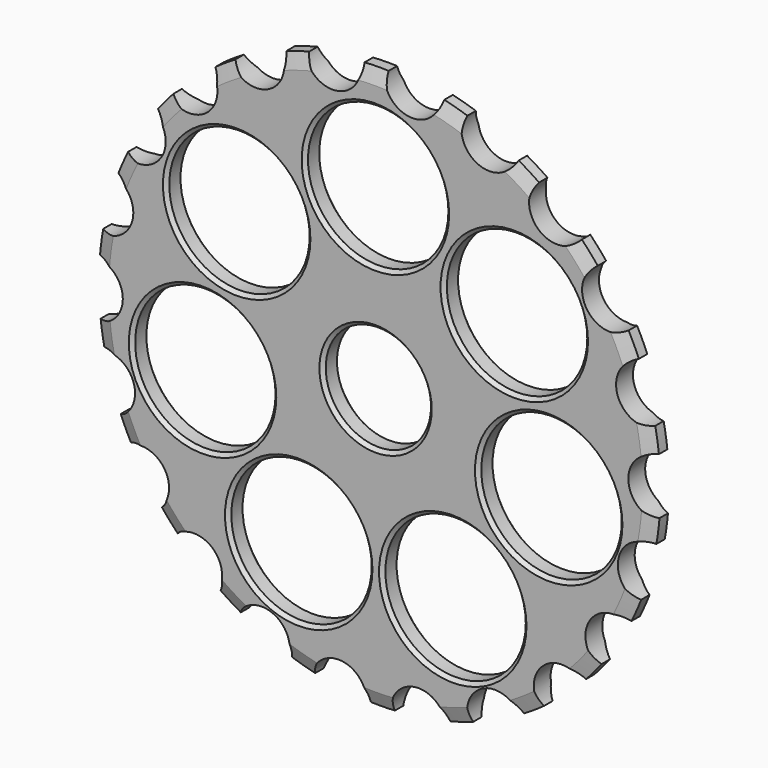
from build123d import *

# Parameters (mm, degrees)
F0_R       = 10
F0_R_2     = 7.5
F1_DEPTH   = 3
F2_SIZE2   = 0.75
F2_SIZE    = 2
F2_2_SIZE2 = 0.75
F2_2_SIZE  = 2
F4_SIZE    = 0.5


# Not quite as in the source:
# - two fillets or chamfers of one size are made in one step


with BuildPart() as f1:
    # F0 (on Front) → F1 (new body)
    with BuildSketch(Plane.XZ):
        with BuildLine():
            ThreePointArc((39.8415623905, -3.556670674), (35.9978191055, 0.3962570459), (39.7536154095, 4.4328390311))
            ThreePointArc((39.7536154095, 4.4328390311), (39.5277999491, 6.1280528053), (39.2297290943, 7.8120647197))
            ThreePointArc((39.2297290943, 7.8120647197), (34.4280159865, 10.5219634686), (36.8944395869, 15.4531656165))
            ThreePointArc((36.8944395869, 15.4531656165), (36.2001743283, 17.0160917546), (35.4397364551, 18.5479130899))
            ThreePointArc((35.4397364551, 18.5479130899), (30.0690597635, 19.7952429876), (31.0462956886, 25.2215686272))
            ThreePointArc((31.0462956886, 25.2215686272), (29.9398258742, 26.5255881485), (28.7786271366, 27.7811198502))
            ThreePointArc((28.7786271366, 27.7811198502), (23.2740871461, 27.4648296466), (22.6829655531, 32.9466701461))
            ThreePointArc((22.6829655531, 32.9466701461), (21.2539307867, 33.8861391444), (19.7860446005, 34.763665501))
            ThreePointArc((19.7860446005, 34.763665501), (14.5935864044, 32.9093791473), (12.4819964492, 38.0026283912))
            ThreePointArc((12.4819964492, 38.0026283912), (10.8461686289, 38.5014366755), (9.190514403, 38.9298657204))
            ThreePointArc((9.190514403, 38.9298657204), (4.7308000836, 35.687806469), (1.2698102264, 39.9798396944))
            ThreePointArc((1.2698102264, 39.9798396944), (-0.4402856066, 39.9975767839), (-2.1495766133, 39.9421997439))
            ThreePointArc((-2.1495766133, 39.9421997439), (-2.1334373815, 39.7352791434), (-2.1280528053, 39.5277999491))
            ThreePointArc((-2.1280528053, 39.5277999491), (-5.7211023511, 35.548554879), (-10.0452484692, 38.7181221548))
            ThreePointArc((-10.0452484692, 38.7181221548), (-11.6910705207, 38.2533510961), (-13.3155217164, 37.7186542896))
            ThreePointArc((-13.3155217164, 37.7186542896), (-13.091663124, 36.9740347316), (-13.0160917546, 36.2001743283))
            ThreePointArc((-13.0160917546, 36.2001743283), (-16.0469778506, 32.3193473235), (-20.5465008752, 34.3196926237))
            ThreePointArc((-20.5465008752, 34.3196926237), (-21.9947144307, 33.4100664039), (-23.4027224406, 32.4393677862))
            ThreePointArc((-23.4027224406, 32.4393677862), (-22.751236361, 31.2643139202), (-22.5255881485, 29.9398258742))
            ThreePointArc((-22.5255881485, 29.9398258742), (-25.0140391592, 26.2364193811), (-29.383197975, 27.1408857034))
            ThreePointArc((-29.383197975, 27.1408857034), (-30.5164773851, 25.860096829), (-31.5939737739, 24.5320366291))
            ThreePointArc((-31.5939737739, 24.5320366291), (-30.338699118, 23.1020837184), (-29.8861391444, 21.2539307867))
            ThreePointArc((-29.8861391444, 21.2539307867), (-31.8629258482, 17.8033354818), (-35.8394431235, 17.7632856364))
            ThreePointArc((-35.8394431235, 17.7632856364), (-36.5659768303, 16.2150960049), (-37.2256692487, 14.637265762))
            ThreePointArc((-37.2256692487, 14.637265762), (-35.2531240591, 13.1803633822), (-34.5014366755, 10.8461686289))
            ThreePointArc((-34.5014366755, 10.8461686289), (-36.0077458606, 7.7186286819), (-39.3921897355, 6.9466098095))
            ThreePointArc((-39.3921897355, 6.9466098095), (-39.6531182989, 5.2564445374), (-39.8415623905, 3.556670674))
            ThreePointArc((-39.8415623905, 3.556670674), (-37.1145178551, 2.3324334944), (-35.9975767839, -0.4402856066))
            ThreePointArc((-35.9975767839, -0.4402856066), (-37.0841728042, -3.1811025014), (-39.7536154095, -4.4328390311))
            ThreePointArc((-39.7536154095, -4.4328390311), (-39.5277999491, -6.1280528053), (-39.2297290943, -7.8120647197))
            ThreePointArc((-39.2297290943, -7.8120647197), (-35.7942366206, -8.536271637), (-34.2533510961, -11.6910705207))
            ThreePointArc((-34.2533510961, -11.6910705207), (-34.979542455, -13.9893692353), (-36.8944395869, -15.4531656165))
            ThreePointArc((-36.8944395869, -15.4531656165), (-36.2001743283, -17.0160917546), (-35.4397364551, -18.5479130899))
            ThreePointArc((-35.4397364551, -18.5479130899), (-31.4249568609, -18.5220583719), (-29.4100664039, -21.9947144307))
            ThreePointArc((-29.4100664039, -21.9947144307), (-29.8424984045, -23.803708231), (-31.0462956886, -25.2215686272))
            ThreePointArc((-31.0462956886, -25.2215686272), (-29.9398258742, -26.5255881485), (-28.7786271366, -27.7811198502))
            ThreePointArc((-28.7786271366, -27.7811198502), (-24.3894033243, -26.7966574143), (-21.860096829, -30.5164773851))
            ThreePointArc((-21.860096829, -30.5164773851), (-22.0713948676, -31.799340374), (-22.6829655531, -32.9466701461))
            ThreePointArc((-22.6829655531, -32.9466701461), (-21.2539307867, -33.8861391444), (-19.7860446005, -34.763665501))
            ThreePointArc((-19.7860446005, -34.763665501), (-15.288757617, -32.674717755), (-12.2150960049, -36.5659768303))
            ThreePointArc((-12.2150960049, -36.5659768303), (-12.2823871279, -37.2965936168), (-12.4819964492, -38.0026283912))
            ThreePointArc((-12.4819964492, -38.0026283912), (-10.8461686289, -38.5014366755), (-9.190514403, -38.9298657204))
            ThreePointArc((-9.190514403, -38.9298657204), (-4.8933188446, -35.6696349324), (-1.2564445374, -39.6531182989))
            ThreePointArc((-1.2564445374, -39.6531182989), (-1.2597873564, -39.8166156321), (-1.2698102264, -39.9798396944))
            ThreePointArc((-1.2698102264, -39.9798396944), (0.4402856066, -39.9975767839), (2.1495766133, -39.9421997439))
            ThreePointArc((2.1495766133, -39.9421997439), (5.5152475248, -35.5750199542), (10.0452484692, -38.7181221548))
            ThreePointArc((10.0452484692, -38.7181221548), (11.6910705207, -38.2533510961), (13.3155217164, -37.7186542896))
            ThreePointArc((13.3155217164, -37.7186542896), (15.3144825791, -32.5801568955), (20.5465008752, -34.3196926237))
            ThreePointArc((20.5465008752, -34.3196926237), (21.9947144307, -33.4100664039), (23.4027224406, -32.4393677862))
            ThreePointArc((23.4027224406, -32.4393677862), (23.8730293337, -26.9458432867), (29.383197975, -27.1408857034))
            ThreePointArc((29.383197975, -27.1408857034), (30.5164773851, -25.860096829), (31.5939737739, -24.5320366291))
            ThreePointArc((31.5939737739, -24.5320366291), (30.49752523, -19.128537708), (35.8394431235, -17.7632856364))
            ThreePointArc((35.8394431235, -17.7632856364), (36.5659768303, -16.2150960049), (37.2256692487, -14.637265762))
            ThreePointArc((37.2256692487, -14.637265762), (34.6512930079, -9.761551766), (39.3921897355, -6.9466098095))
            ThreePointArc((39.3921897355, -6.9466098095), (39.6531182989, -5.2564445374), (39.8415623905, -3.556670674))
        make_face()
        with Locations((-10.9472820638, -22.7902135457)):
            Circle(F0_R, mode=Mode.SUBTRACT)
        with Locations((-24.6436251671, -5.6505359631)):
            Circle(F0_R, mode=Mode.SUBTRACT)
        with Locations((10.9925877174, -22.7683954929)):
            Circle(F0_R, mode=Mode.SUBTRACT)
        with Locations((24.6548147394, -5.6015112432)):
            Circle(F0_R, mode=Mode.SUBTRACT)
        Circle(F0_R_2, mode=Mode.SUBTRACT)
        with Locations((-19.7828158812, 15.7441104498)):
            Circle(F0_R, mode=Mode.SUBTRACT)
        with Locations((-0.0251427409, 25.2831205726)):
            Circle(F0_R, mode=Mode.SUBTRACT)
        with Locations((19.7514633961, 15.7834252226)):
            Circle(F0_R, mode=Mode.SUBTRACT)
    extrude(amount=F1_DEPTH)

    # F2
    f2_edges = [f1.edges().sort_by_distance(p)[0] for p in [
        (-10.846169, 0, -38.501437),
        (-21.253931, 0, -33.886139),
        (-29.939826, 0, -26.525588),
        (-36.200174, 0, -17.016092),
        (-39.5278, 0, -6.128053),
        (-39.653118, 0, 5.256445),
        (-36.565977, 0, 16.215096),
        (-30.516477, 0, 25.860097),
        (-21.994714, 0, 33.410066),
        (-11.691071, 0, 38.253351),
        (-0.440286, 0, 39.997577),
        (10.846169, 0, 38.501437),
        (21.253931, 0, 33.886139),
        (29.939826, 0, 26.525588),
        (36.200174, 0, 17.016092),
        (39.5278, 0, 6.128053),
        (39.653118, 0, -5.256445),
        (36.565977, 0, -16.215096),
        (30.516477, 0, -25.860097),
        (21.994714, 0, -33.410066),
        (11.691071, 0, -38.253351),
        (0.440286, 0, -39.997577),
    ]]
    f2_side = f1.faces().sort_by_distance((-10.54, 0, -37.414606))[0]
    chamfer(f2_edges, length=F2_SIZE, length2=F2_SIZE2, reference=f2_side)

    # F2#2
    f2_2_edges = [f1.edges().sort_by_distance(p)[0] for p in [
        (-10.846169, -3, -38.501437),
        (0.440286, -3, -39.997577),
        (11.691071, -3, -38.253351),
        (21.994714, -3, -33.410066),
        (30.516477, -3, -25.860097),
        (36.565977, -3, -16.215096),
        (39.653118, -3, -5.256445),
        (39.5278, -3, 6.128053),
        (36.200174, -3, 17.016092),
        (29.939826, -3, 26.525588),
        (21.253931, -3, 33.886139),
        (10.846169, -3, 38.501437),
        (-0.440286, -3, 39.997577),
        (-11.691071, -3, 38.253351),
        (-21.994714, -3, 33.410066),
        (-30.516477, -3, 25.860097),
        (-36.565977, -3, 16.215096),
        (-39.653118, -3, 5.256445),
        (-39.5278, -3, -6.128053),
        (-36.200174, -3, -17.016092),
        (-29.939826, -3, -26.525588),
        (-21.253931, -3, -33.886139),
    ]]
    f2_2_side = f1.faces().sort_by_distance((-10.54, -3, -37.414606))[0]
    chamfer(f2_2_edges, length=F2_2_SIZE, length2=F2_2_SIZE2, reference=f2_2_side)

    # F4
    f4_edges = [f1.edges().sort_by_distance(p)[0] for p in [
        (-7.5, -3, 0),
        (-7.5, 0, 0),
        (-10.025143, -3, 25.283121),
        (9.751463, -3, 15.783425),
        (14.654815, -3, -5.601511),
        (0.992588, -3, -22.768395),
        (-20.947282, -3, -22.790214),
        (-34.643625, -3, -5.650536),
        (-29.782816, -3, 15.74411),
        (-10.025143, 0, 25.283121),
        (9.751463, 0, 15.783425),
        (14.654815, 0, -5.601511),
        (0.992588, 0, -22.768395),
        (-20.947282, 0, -22.790214),
        (-34.643625, 0, -5.650536),
        (-29.782816, 0, 15.74411),
    ]]
    chamfer(f4_edges, length=F4_SIZE)


solid = f1.part
